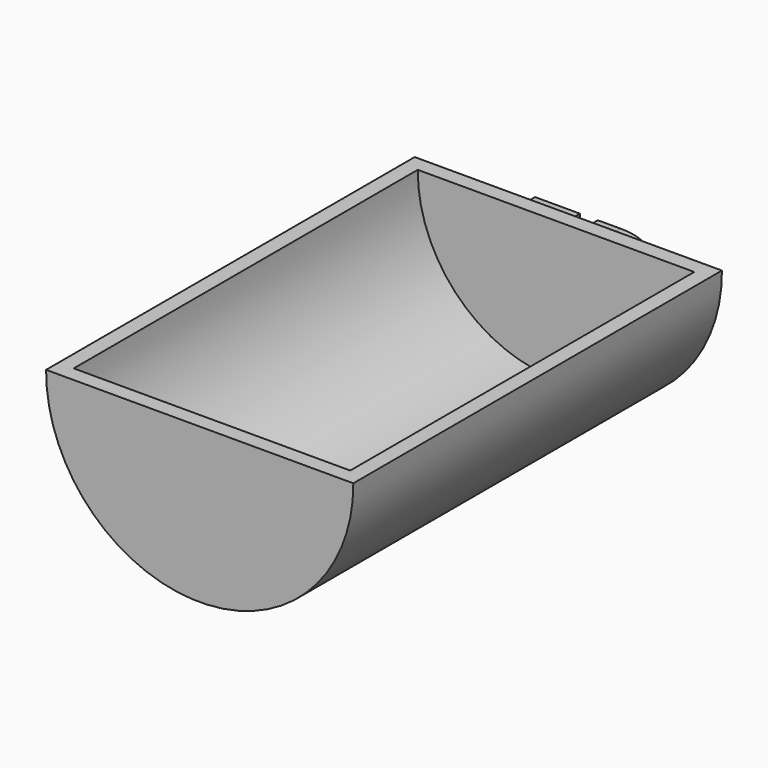
from build123d import *

# Parameters (mm, degrees)
F1_DEPTH     = 76.2
F2_T         = -2.54
F3_TEXT_SIZE = 18.6560235711
F4_DEPTH     = 5.08


# Not quite as in the source:
# - Text() gives the source's letters only with a copy of the font that has no kerning and outlines rounded to 1/6400 em; it was checked with that copy


with BuildPart() as f1:
    # F0 (on Front) → F1 (new body)
    with BuildSketch(Plane.XZ):
        with BuildLine():
            Line((-40.1510037482, 43.9424648225), (-65.555639565, 43.9424648225))
            ThreePointArc((-65.555639565, 43.9424648225), (-40.1510037482, 18.3801199337), (-14.7463679314, 43.9424648225))
            Line((-14.7463679314, 43.9424648225), (-40.1510037482, 43.9424648225))
        make_face()
    extrude(amount=F1_DEPTH)

    # F2
    f2_openings = [f1.faces().sort_by_distance(p)[0] for p in [
        (-40.151004, -38.1, 43.942465),
    ]]
    offset(amount=F2_T, openings=f2_openings)

    # F3 (on Front) → F4 (join)
    with BuildSketch(Plane.XZ):
        with Locations((-51.5392888337, 27.8866980225)):
            Text('EB', F3_TEXT_SIZE, font='Open Sans', text_align=(TextAlign.LEFT, TextAlign.BOTTOM))
    extrude(amount=-F4_DEPTH)


solid = f1.part
